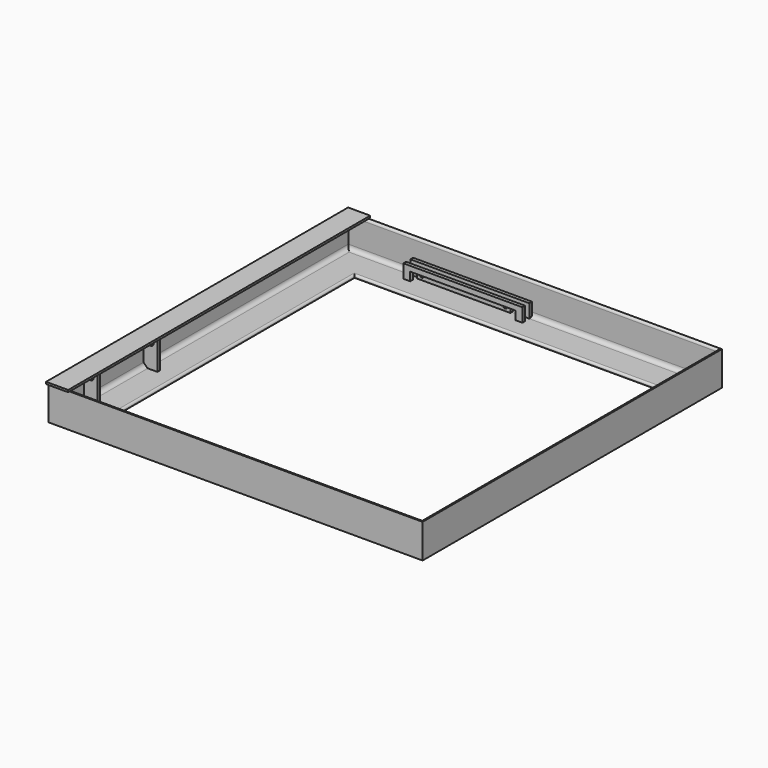
from build123d import *

# Parameters (mm, degrees)
F5_R      = 9
F6_DEPTH  = 10
F9_W      = 65
F9_H      = 1110
F10_DEPTH = 6
F12_W     = 275
F12_H     = 25
F12_R     = 6
F13_DEPTH = 10
F16_DEPTH = 10
F19_DEPTH = 10


with BuildPart() as f2:
    # F2: sweep along a path in F0
    with BuildLine(Plane.XY) as f2_path:
        Line((0, 0), (0, 1100))
        Line((0, 1100), (1100, 1100))
        Line((1100, 1100), (1100, 0))
        Line((1100, 0), (0, 0))
    # F1 (on Front) → F2 (sweep)
    with BuildSketch(Plane.XZ):
        with BuildLine():
            Line((2, 0), (0, 0))
            Line((0, 0), (0, -100))
            Line((0, -100), (100, -100))
            Line((100, -100), (100, -98))
            ThreePointArc((100, -98), (98.2426406871, -93.7573593129), (94, -92))
            Line((94, -92), (20, -92))
            ThreePointArc((20, -92), (11.5147186258, -88.4852813742), (8, -80))
            Line((8, -80), (8, -6))
            ThreePointArc((8, -6), (6.2426406871, -1.7573593129), (2, 0))
        make_face()
    sweep(path=f2_path.line, transition=Transition.RIGHT)


with BuildPart() as f6:
    # F5 (on line) → F6 (new body)
    with BuildSketch(Plane(origin=(0, 120, 0), x_dir=(-1, 0, 0), z_dir=(0, 1, 0))):
        Polygon((-48, 0), (-48, -92), (-18.9421893259, -92), (-8, -81.0578106741), (-8, 0), align=None)
        with Locations((-28, -22)):
            Circle(F5_R, mode=Mode.SUBTRACT)
    extrude(amount=F6_DEPTH)


with BuildPart() as f7_1:
    # F7: copy of F6
    add(f6.part.moved(Location((0, 220, 0))))


with BuildPart() as f10:
    # F9 (on face) → F10 (new body)
    with BuildSketch(Plane.XY):
        with Locations((29.5, 550)):
            Rectangle(F9_W, F9_H)
    extrude(amount=F10_DEPTH)


with BuildPart() as f13:
    # F12 (on face) → F13 (new body)
    with BuildSketch(Plane(origin=(0, 1060, 0), x_dir=(-1, 0, 0), z_dir=(0, 1, 0))):
        with Locations((-372.5, -69.5)):
            Rectangle(F12_W, F12_H)
        with Locations((-495, -69.5)):
            Circle(F12_R, mode=Mode.SUBTRACT)
        with Locations((-250, -69.5)):
            Circle(F12_R, mode=Mode.SUBTRACT)
    extrude(amount=F13_DEPTH)


with BuildPart() as f16:
    # F15 (on face) → F16 (new body)
    with BuildSketch(Plane(origin=(0, 1080, 0), x_dir=(-1, 0, 0), z_dir=(0, 1, 0))):
        Polygon((-220, -92), (-200, -92), (-200, -52), (-550, -52), (-550, -92), (-530, -92), (-530, -67), (-220, -67), align=None)
    extrude(amount=F16_DEPTH)


with BuildPart() as f19:
    # F18 (on face) → F19 (new body)
    with BuildSketch(Plane(origin=(0, 1054.384, 0), x_dir=(-1, 0, 0), z_dir=(0, 1, 0))):
        Polygon((-220, -92), (-200, -92), (-200, -52), (-550, -52), (-550, -92), (-530, -92), (-530, -67), (-220, -67), align=None)
    extrude(amount=F19_DEPTH)


solid = Compound([f2.part, f6.part, f7_1.part, f10.part, f13.part, f16.part, f19.part])
